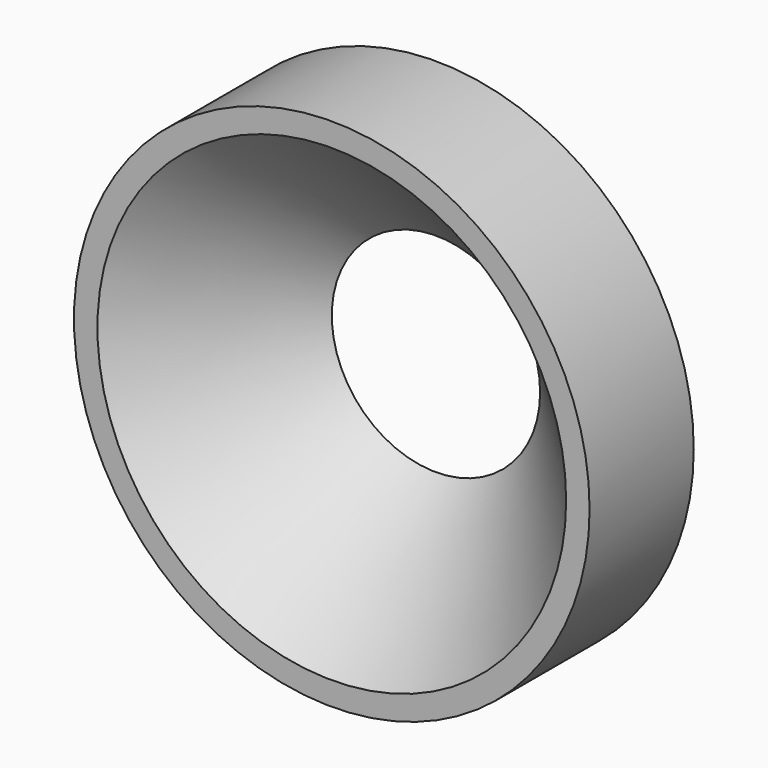
from build123d import *

# Parameters (mm, degrees)
F0_R     = 4.95
F0_R_2   = 3.85
F0_R_3   = 2
F1_DEPTH = 2.5
F2_DEPTH = 3.19
F3_SIZE2 = 2.49999
F3_SIZE  = 2.49999


# Not quite as in the source:
# - a fillet or chamfer is up to 0.001 mm smaller than in the source, because OpenCascade refuses the exact size


with BuildPart() as f1:
    # F0 (on Front) → F1 (new body)
    with BuildSketch(Plane.XZ):
        Circle(F0_R)
        Circle(F0_R_2, mode=Mode.SUBTRACT)
        Circle(F0_R_2)
        Circle(F0_R_3, mode=Mode.SUBTRACT)
        Circle(F0_R_3)
    extrude(amount=F1_DEPTH)

    # F0 (on Front) → F2 (cut)
    with BuildSketch(Plane.XZ):
        Circle(F0_R_3)
    extrude(amount=F2_DEPTH, mode=Mode.SUBTRACT)

    # F3 (size 2.5 and 2.5 in the source; OpenCascade refuses exactly that, so slightly less here)
    f3_edges = [f1.edges().sort_by_distance(p)[0] for p in [
        (-2, -2.5, 0),
    ]]
    chamfer(f3_edges, length=F3_SIZE, length2=F3_SIZE2)


solid = f1.part
